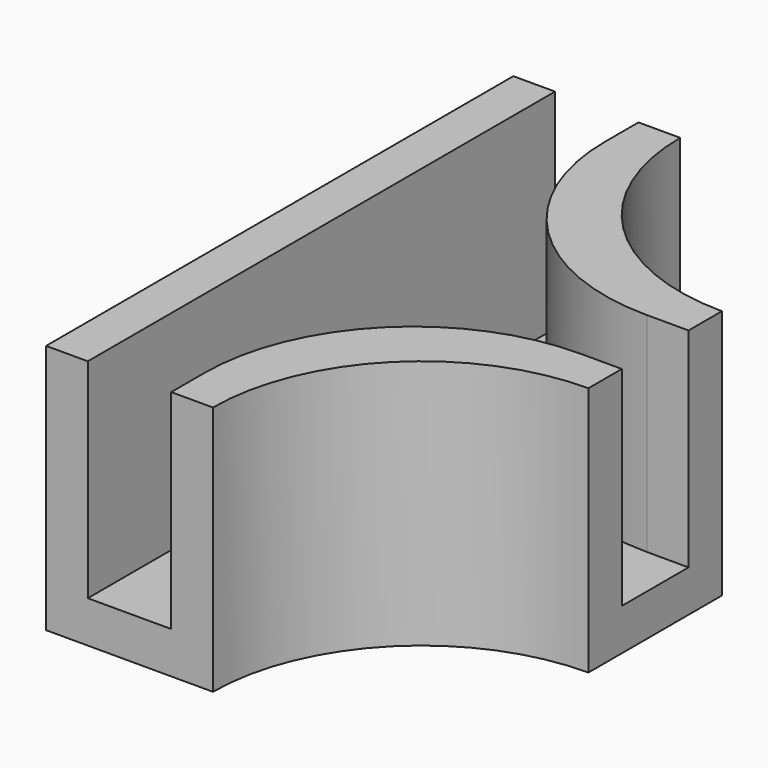
from build123d import *

# Parameters (mm, degrees)
F0_W     = 5
F0_H     = 4
F1_DEPTH = 1
F2_W     = 1
F2_H     = 5
F3_DEPTH = 5
F4_R     = 4.99999
F2_H_2   = 14
F5_DEPTH = 5


# Not quite as in the source:
# - a fillet or chamfer is up to 0.001 mm smaller than in the source, because OpenCascade refuses the exact size


with BuildPart() as f1:
    # F0 (on Top) → F1 (new body)
    with BuildSketch(Plane.XY):
        Polygon((-4.5, -7), (-0.5, -7), (-0.5, -2), (-0.5, 2), (-0.5, 7), (-4.5, 7), align=None)
        with Locations((2, 0)):
            Rectangle(F0_W, F0_H)
    extrude(amount=F1_DEPTH)

    # F2 (on face) → F3 (join)
    with BuildSketch(Plane.XY.offset(1)):
        Polygon((-0.5, -2), (4.5, -2), (4.5, -1), (-1.5, -1), (-1.5, -2), align=None)
        with Locations((-1, -4.5)):
            Rectangle(F2_W, F2_H)
        Polygon((-1.5, 1), (4.5, 1), (4.5, 2), (-0.5, 2), (-1.5, 2), align=None)
        with Locations((-1, 4.5)):
            Rectangle(F2_W, F2_H)
    extrude(amount=F3_DEPTH)

    # F4 (radius 5 in the source; OpenCascade refuses exactly that, so slightly less here)
    f4_edges = [f1.edges().sort_by_distance(p)[0] for p in [
        (-0.5, -2, 3),
        (-1.5, 1, 3.5),
        (-1.5, -1, 3.5),
        (-0.5, 2, 3),
    ]]
    fillet(f4_edges, radius=F4_R)

    # F2 (on face) → F5 (join)
    with BuildSketch(Plane.XY.offset(1)):
        with Locations((-4, 0)):
            Rectangle(F2_W, F2_H_2)
    extrude(amount=F5_DEPTH)


solid = f1.part
